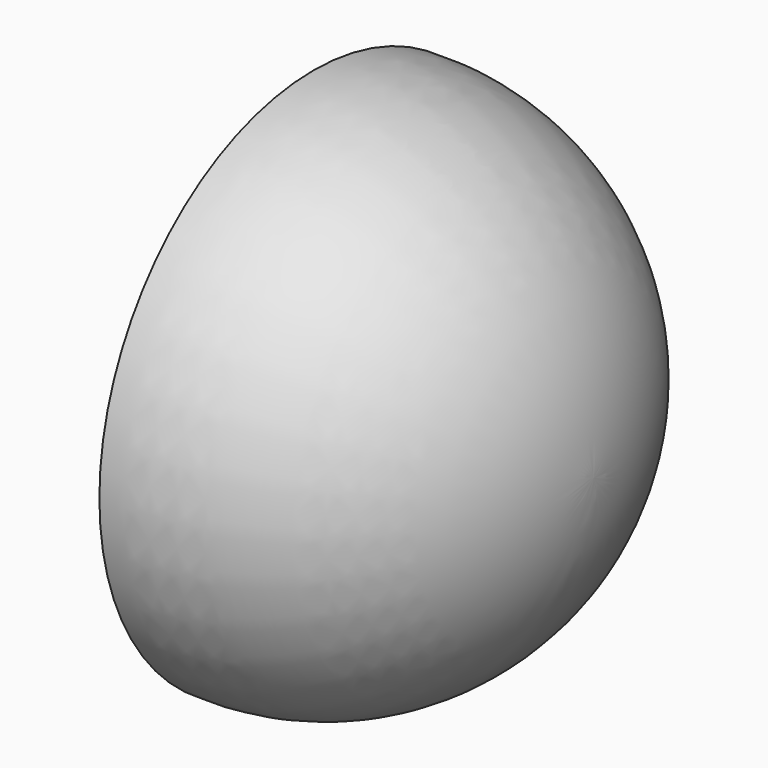
from build123d import *

# Parameters (mm, degrees)
F7_DEPTH  = 2.5
F13_DEPTH = 2
F49_DEPTH = 2
F54_R     = 0.6074168768
F55_DEPTH = 20
F56_R     = 1.0752530324
F57_DEPTH = 25


# Not quite as in the source:
# - ends of sketch curves that miss each other by under 0.0002 mm in the source are joined
# - the program builds the solid bodies; features that only make, move or delete a surface that nothing else refers to are left out


with BuildPart() as f1:
    # F0 (on Front) → F1 (revolve)
    with BuildSketch(Plane.XZ):
        with BuildLine():
            Line((0, 20), (0, 0))
            Line((0, 0), (20.9032140208, 0))
            ThreePointArc((20.9032140208, 0), (14.7145025663, 14.4554109076), (0, 20))
        make_face()
    revolve(axis=Axis((10.4516070104, 0, 0), (1, 0, 0)))

    # F2 (on Right) → F3 (revolve)
    with BuildSketch(Plane.YZ):
        with BuildLine():
            Line((-3, 0), (0, 0))
            Line((0, 0), (0, 3))
            ThreePointArc((0, 3), (-2.1378188048, 2.1378188048), (-3, 0))
        make_face()
    revolve(axis=Axis((0, -1.5, 0), (0, -1, 0)))

    # F4 (on face) → F5 (revolve)
    with BuildSketch(Plane(origin=(0, 0, 0), x_dir=(0, -1, 0), z_dir=(-1, 0, 0))):
        with BuildLine():
            Line((-3, 0), (0, 0))
            Line((0, 0), (0, 3))
            ThreePointArc((0, 3), (-2.1060516761, 2.1060516761), (-3, 0))
        make_face()
    revolve(axis=Axis((0, 1.5, 0), (0, 1, 0)))

    # F20 (on face) → F21 (revolve)
    with BuildSketch(Plane(origin=(0, 0, 0), x_dir=(0, -1, 0), z_dir=(-1, 0, 0))):
        with BuildLine():
            ThreePointArc((-7.6594431885, -3.8764923811), (-8.2749807984, -4.5285373926), (-7.6594431885, -5.1805824041))
            Line((-7.6594431885, -5.1805824041), (-7.6594431885, -3.8764923811))
        make_face()
    revolve(axis=Axis((0, 7.6594431885, -4.5285373926), (0, 0, 1)))

    # F22 (on face) → F23 (revolve)
    with BuildSketch(Plane(origin=(0, 0, 0), x_dir=(0, -1, 0), z_dir=(-1, 0, 0))):
        with BuildLine():
            ThreePointArc((12.7418441698, 5.2346289158), (12.1728994386, 4.6591833234), (12.7418441698, 4.083737731))
            Line((12.7418441698, 4.083737731), (12.7418441698, 5.2346289158))
        make_face()
    revolve(axis=Axis((0, -12.7418441698, 4.6591833234), (0, 0, 1)))

    # F24 (on face) → F25 (revolve)
    with BuildSketch(Plane(origin=(0, 0, 0), x_dir=(0, -1, 0), z_dir=(-1, 0, 0))):
        with BuildLine():
            ThreePointArc((-5.9676826932, -12.5175017115), (-6.7753176022, -13.3251366206), (-5.9676826932, -14.1327715296))
            Line((-5.9676826932, -14.1327715296), (-5.9676826932, -12.5175017115))
        make_face()
    revolve(axis=Axis((0, 5.9676826932, -13.3251366206), (0, 0, 1)))

    # F26 (on face) → F27 (revolve)
    with BuildSketch(Plane(origin=(0, 0, 0), x_dir=(0, -1, 0), z_dir=(-1, 0, 0))):
        with BuildLine():
            ThreePointArc((-2.6682941243, 17.2478277236), (-3.8004852056, 17.2364370857), (-3.7481172476, 16.1054003984))
            Line((-3.7481172476, 16.1054003984), (-2.6682941243, 17.2478277236))
        make_face()
    revolve(axis=Axis((0, 3.208205686, 16.676614061), (0, -0.6869139736, 0.7267387377)))

    # F30 (on face) → F31 (revolve)
    with BuildSketch(Plane(origin=(0, 0, 0), x_dir=(0, -1, 0), z_dir=(-1, 0, 0))):
        with BuildLine():
            ThreePointArc((2.065625973, 2.9552876949), (1.8622744828, 3.1655695777), (1.6589229926, 2.9552876949))
            Line((1.6589229926, 2.9552876949), (2.065625973, 2.9552876949))
        make_face()
    revolve(axis=Axis((0, -1.8622744828, 2.9552876949), (0, -1, 0)))

    # F32 (on face) → F33 (revolve)
    with BuildSketch(Plane(origin=(0, 0, 0), x_dir=(0, -1, 0), z_dir=(-1, 0, 0))):
        with BuildLine():
            ThreePointArc((4.7333193943, 2.0018331707), (4.6435543336, 2.0690382814), (4.5537892729, 2.0018331707))
            Line((4.5537892729, 2.0018331707), (4.7333193943, 2.0018331707))
        make_face()
    revolve(axis=Axis((0, -4.6435543336, 2.0018331707), (0, -1, 0)))

    # F34 (on face) → F35 (revolve)
    with BuildSketch(Plane(origin=(0, 0, 0), x_dir=(0, -1, 0), z_dir=(-1, 0, 0))):
        with BuildLine():
            Line((4.7080395743, -0.380108133), (4.4907717966, -0.380108133))
            ThreePointArc((4.4907717966, -0.380108133), (4.5994056854, -0.4801378843), (4.7080395743, -0.380108133))
        make_face()
    revolve(axis=Axis((0, -4.5994056854, -0.380108133), (0, -1, 0)))

    # F36 (on face) → F37 (revolve)
    with BuildSketch(Plane(origin=(0, 0, 0), x_dir=(0, -1, 0), z_dir=(-1, 0, 0))):
        with BuildLine():
            ThreePointArc((2.4876960088, -3.15255858), (2.3429562571, -2.9939137255), (2.1982165053, -3.15255858))
            Line((2.1982165053, -3.15255858), (2.4876960088, -3.15255858))
        make_face()
    revolve(axis=Axis((0, -2.3429562571, -3.15255858), (0, -1, 0)))

    # F38 (on face) → F39 (revolve)
    with BuildSketch(Plane(origin=(0, 0, 0), x_dir=(0, -1, 0), z_dir=(-1, 0, 0))):
        with BuildLine():
            ThreePointArc((3.7825170439, 0.9611435235), (3.6940083373, 1.0506368525), (3.6054996308, 0.9611435235))
            Line((3.6054996308, 0.9611435235), (3.7825170439, 0.9611435235))
        make_face()
    revolve(axis=Axis((0, -3.6940083373, 0.9611435235), (0, -1, 0)))

    # F40 (on face) → F41 (revolve)
    with BuildSketch(Plane(origin=(0, 0, 0), x_dir=(0, -1, 0), z_dir=(-1, 0, 0))):
        with BuildLine():
            ThreePointArc((0.5645051133, 3.9112772793), (0.4595427308, 4.0212758064), (0.3545803484, 3.9112772793))
            Line((0.3545803484, 3.9112772793), (0.5645051133, 3.9112772793))
        make_face()
    revolve(axis=Axis((0, -0.4595427308, 3.9112772793), (0, -1, 0)))

    # F42 (on face) → F43 (revolve)
    with BuildSketch(Plane(origin=(0, 0, 0), x_dir=(0, -1, 0), z_dir=(-1, 0, 0))):
        with BuildLine():
            ThreePointArc((5.4294881411, 0.7984926924), (5.4440247442, 1.0004788431), (5.2415728569, 1.005269587))
            Line((5.2415728569, 1.005269587), (5.4294881411, 0.7984926924))
        make_face()
    revolve(axis=Axis((0, -5.335530499, 0.9018811397), (0, -0.6725479403, -0.7400535575)))

    # F44 (on face) → F45 (revolve)
    with BuildSketch(Plane(origin=(0, 0, 0), x_dir=(0, -1, 0), z_dir=(-1, 0, 0))):
        with BuildLine():
            ThreePointArc((4.5250565745, -1.9389539957), (4.3312804717, -1.9511606938), (4.3379967101, -2.1452046931))
            Line((4.3379967101, -2.1452046931), (4.5250565745, -1.9389539957))
        make_face()
    revolve(axis=Axis((0, -4.4315266423, -2.0420793444), (0, -0.6718056347, 0.740727473)))

    # F46 (on face) → F47 (revolve)
    with BuildSketch(Plane(origin=(0, 0, 0), x_dir=(0, -1, 0), z_dir=(-1, 0, 0))):
        with BuildLine():
            Line((3.5201823339, -1.579977572), (3.3489386551, -1.579977572))
            ThreePointArc((3.3489386551, -1.579977572), (3.4345604945, -1.668621835), (3.5201823339, -1.579977572))
        make_face()
    revolve(axis=Axis((0, -3.4345604945, -1.579977572), (0, -1, 0)))

    # F52 (on face) → F53 (revolve)
    with BuildSketch(Plane(origin=(0, 0, 0), x_dir=(0, -1, 0), z_dir=(-1, 0, 0))):
        with BuildLine():
            ThreePointArc((2.2028738167, -10.7880309224), (1.6207013978, -10.2191004003), (1.0385289788, -10.7880309224))
            Line((1.0385289788, -10.7880309224), (2.2028738167, -10.7880309224))
        make_face()
    revolve(axis=Axis((0, -1.6207013978, -10.7880309224), (0, -1, 0)))

    # F54 (on face) → F55 (cut)
    with BuildSketch(Plane(origin=(0, 0, 0), x_dir=(0, -1, 0), z_dir=(-1, 0, 0))):
        with Locations((2.1903119247, -18.6780034797)):
            Circle(F54_R)
    extrude(amount=F55_DEPTH, mode=Mode.SUBTRACT)

    # F56 (on face) → F57 (cut)
    with BuildSketch(Plane(origin=(0, 0, 0), x_dir=(0, -1, 0), z_dir=(-1, 0, 0))):
        with Locations((2.9139111284, -17.4465067685)):
            Circle(F56_R)
    extrude(amount=-F57_DEPTH, mode=Mode.SUBTRACT)


with BuildPart() as f7:
    # F6 (on face) → F7 (new body)
    with BuildSketch(Plane(origin=(0, 0, 0), x_dir=(0, -1, 0), z_dir=(-1, 0, 0))):
        with BuildLine():
            add(Edge.make_bspline(
                [(13.0212418735, -3.58440727), (10.7913677509, -1.6396786361), (6.5594301058, -8.7429022088), (2.3274924606, -15.8461257815), (8.7893042283, -10.6876308427), (15.2511159961, -5.5291359038), (13.0212418735, -3.58440727)],
                knots=[0, 0, 0, 2.0943951024, 2.0943951024, 4.1887902048, 4.1887902048, 6.2831853072, 6.2831853072, 6.2831853072], degree=2, weights=[1, 0.5, 1, 0.5, 1, 0.5, 1]))
        make_face()
    extrude(amount=F7_DEPTH)


with BuildPart() as f13:
    # F12 (on face) → F13 (new body)
    with BuildSketch(Plane(origin=(0, 0, 0), x_dir=(0, -1, 0), z_dir=(-1, 0, 0))):
        with BuildLine():
            add(Edge.make_bspline(
                [(10.9271379188, 7.5598936528), (12.4094731309, 10.030454188), (5.7548497871, 12.3432447088), (-0.8997735567, 14.6560352296), (4.2725145749, 9.8726841736), (9.4448027066, 5.0893331176), (10.9271379188, 7.5598936528)],
                knots=[0, 0, 0, 2.0943951024, 2.0943951024, 4.1887902048, 4.1887902048, 6.2831853072, 6.2831853072, 6.2831853072], degree=2, weights=[1, 0.5, 1, 0.5, 1, 0.5, 1]))
        make_face()
    extrude(amount=F13_DEPTH)


with BuildPart() as f29:
    # F28 (on face) → F29 (revolve)
    with BuildSketch(Plane(origin=(0, 0, 0), x_dir=(0, -1, 0), z_dir=(-1, 0, 0))):
        with BuildLine():
            ThreePointArc((3.4040999599, 3.4889467061), (3.2618925907, 3.612536586), (3.1196852215, 3.4889467061))
            Line((3.1196852215, 3.4889467061), (3.4040999599, 3.4889467061))
        make_face()
    revolve(axis=Axis((0, -3.2618925907, 3.4889467061), (0, -1, 0)))


with BuildPart() as f49:
    # F48 (on face) → F49 (new body)
    with BuildSketch(Plane(origin=(0, 0, 0), x_dir=(0, -1, 0), z_dir=(-1, 0, 0))):
        with BuildLine():
            add(Edge.make_bspline(
                [(-12.8653030843, -4.054680001), (-15.7865357239, -4.054680001), (-14.3259194041, -9.1504866723), (-12.8653030843, -14.2462933436), (-11.4046867644, -9.1504866723), (-9.9440704446, -4.054680001), (-12.8653030843, -4.054680001)],
                knots=[0, 0, 0, 2.0943951024, 2.0943951024, 4.1887902048, 4.1887902048, 6.2831853072, 6.2831853072, 6.2831853072], degree=2, weights=[1, 0.5, 1, 0.5, 1, 0.5, 1]))
        make_face()
    extrude(amount=F49_DEPTH)


solid = Compound([f1.part, f7.part, f13.part, f29.part, f49.part])
